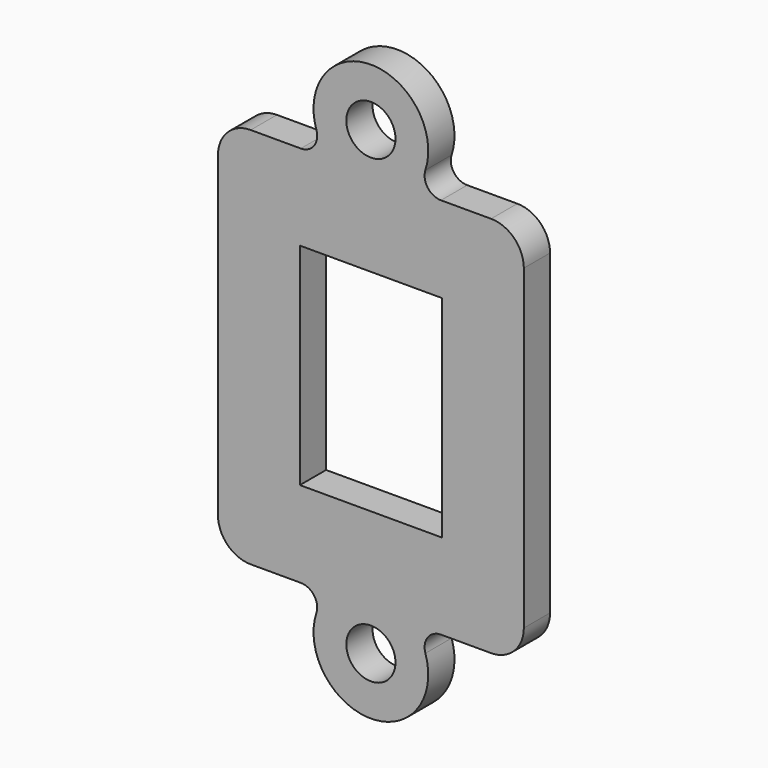
from build123d import *

# Parameters (mm, degrees)
F0_R     = 2.25
F0_W     = 13
F0_H     = 19.3
F1_DEPTH = 3


# Not quite as in the source:
# - a feature names something its author has since deleted; it is built from what else it names


with BuildPart() as f1:
    # F0 (on Front) → F1 (new body)
    with BuildSketch(Plane.XZ):
        with BuildLine():
            Line((-6.4150214341, 17.5), (-11, 17.5))
            ThreePointArc((-11, 17.5), (-13.1213203436, 16.6213203436), (-14, 14.5))
            Line((-14, 14.5), (-14, -14.5))
            ThreePointArc((-14, -14.5), (-13.1213203436, -16.6213203436), (-11, -17.5))
            Line((-11, -17.5), (-6.4150214341, -17.5))
            ThreePointArc((-6.4150214341, -17.5), (-5.200525654, -18.1196591569), (-4.9894611154, -19.4666666667))
            ThreePointArc((-4.9894611154, -19.4666666667), (0, -26.35), (4.9894611154, -19.4666666667))
            ThreePointArc((4.9894611154, -19.4666666667), (5.200525654, -18.1196591569), (6.4150214341, -17.5))
            Line((6.4150214341, -17.5), (11, -17.5))
            ThreePointArc((11, -17.5), (13.1213203436, -16.6213203436), (14, -14.5))
            Line((14, -14.5), (14, 14.5))
            ThreePointArc((14, 14.5), (13.1213203436, 16.6213203436), (11, 17.5))
            Line((11, 17.5), (6.4150214341, 17.5))
            ThreePointArc((6.4150214341, 17.5), (5.200525654, 18.1196591569), (4.9894611154, 19.4666666667))
            ThreePointArc((4.9894611154, 19.4666666667), (0, 26.35), (-4.9894611154, 19.4666666667))
            ThreePointArc((-4.9894611154, 19.4666666667), (-5.200525654, 18.1196591569), (-6.4150214341, 17.5))
        make_face()
        with Locations((0, -21.1)):
            Circle(F0_R, mode=Mode.SUBTRACT)
        Rectangle(F0_W, F0_H, mode=Mode.SUBTRACT)
        with Locations((0, 21.1)):
            Circle(F0_R, mode=Mode.SUBTRACT)
    extrude(amount=F1_DEPTH)


solid = f1.part
